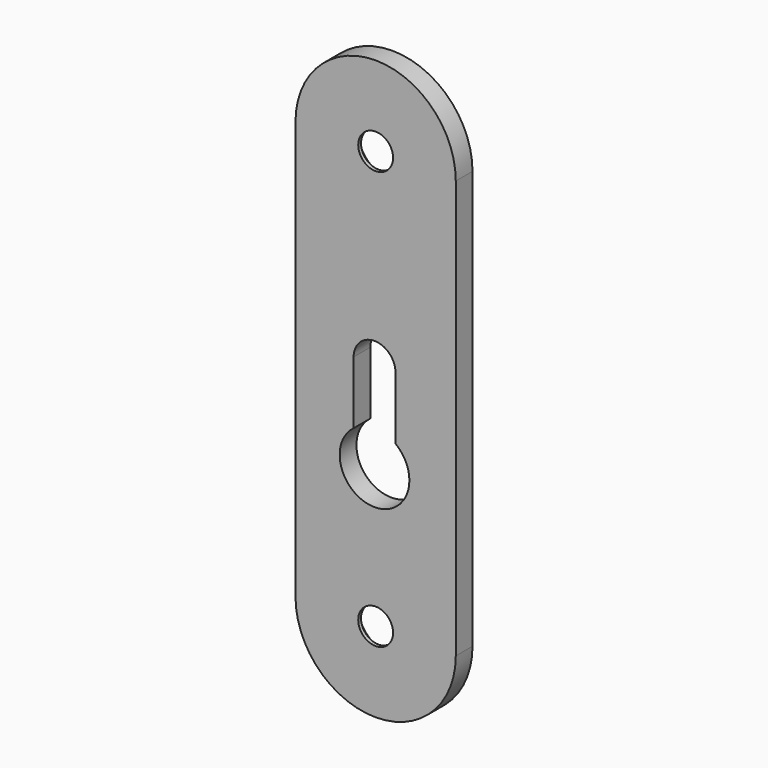
from build123d import *

# Parameters (mm, degrees)
F0_W           = 11.5
F0_H           = 30
F1_DEPTH       = 1.5
F2_D           = 2.5
F2_CSINK_D     = 5
F2_CSINK_ANGLE = 90
F4_DEPTH       = 25
F5_R           = 1.49999


# Not quite as in the source:
# - a fillet or chamfer is up to 0.001 mm smaller than in the source, because OpenCascade refuses the exact size


with BuildPart() as f1:
    # F0 (on Front) → F1 (new body)
    with BuildSketch(Plane.XZ):
        with BuildLine():
            ThreePointArc((-3.8116748205, 37.8448306397), (-9.5616748205, 43.5948306397), (-15.3116748205, 37.8448306397))
            Line((-15.3116748205, 37.8448306397), (-3.8116748205, 37.8448306397))
        make_face()
        with Locations((-9.5616748205, 22.8448306397)):
            Rectangle(F0_W, F0_H)
        with BuildLine():
            Line((-3.8116748205, 7.8448306397), (-15.3116748205, 7.8448306397))
            ThreePointArc((-15.3116748205, 7.8448306397), (-9.5616748205, 2.0948306397), (-3.8116748205, 7.8448306397))
        make_face()
    extrude(amount=F1_DEPTH)

    # F2 (through all)
    with Locations(Plane(origin=(0, 0, 0), x_dir=(1, 0, 0), z_dir=(0, 1, 0))):
        with Locations((-9.5616748205, -37.8448306397), (-9.5616748205, -7.8448306397)):
            CounterSinkHole(F2_D / 2, F2_CSINK_D / 2, counter_sink_angle=F2_CSINK_ANGLE)

    # F3 (on face) → F4 (cut)
    with BuildSketch(Plane.XZ):
        with BuildLine():
            Line((-8.1408721001, 19.8448306397), (-8.1408721001, 25.8448306397))
            Line((-8.1408721001, 25.8448306397), (-11.1408721001, 25.8448306397))
            Line((-11.1408721001, 25.8448306397), (-11.1408721001, 19.8448306397))
            ThreePointArc((-11.1408721001, 19.8448306397), (-9.6408721001, 20.3448306397), (-8.1408721001, 19.8448306397))
        make_face()
        with BuildLine():
            ThreePointArc((-7.1408721001, 17.8448306397), (-7.4048041226, 18.9628646284), (-8.1408721001, 19.8448306397))
            Line((-8.1408721001, 19.8448306397), (-8.1408721001, 17.8448306397))
            Line((-8.1408721001, 17.8448306397), (-11.1408721001, 17.8448306397))
            Line((-11.1408721001, 17.8448306397), (-11.1408721001, 19.8448306397))
            ThreePointArc((-11.1408721001, 19.8448306397), (-10.7589060888, 15.6087626622), (-7.1408721001, 17.8448306397))
        make_face()
        with BuildLine():
            Line((-8.1408721001, 17.8448306397), (-8.1408721001, 19.8448306397))
            ThreePointArc((-8.1408721001, 19.8448306397), (-9.6408721001, 20.3448306397), (-11.1408721001, 19.8448306397))
            Line((-11.1408721001, 19.8448306397), (-11.1408721001, 17.8448306397))
            Line((-11.1408721001, 17.8448306397), (-8.1408721001, 17.8448306397))
        make_face()
    extrude(amount=F4_DEPTH, mode=Mode.SUBTRACT)

    # F5 (radius 1.5 in the source; OpenCascade refuses exactly that, so slightly less here)
    f5_edges = [f1.edges().sort_by_distance(p)[0] for p in [
        (-8.140872, -0.75, 25.844831),
        (-11.140872, -0.75, 25.844831),
    ]]
    fillet(f5_edges, radius=F5_R)


solid = f1.part
